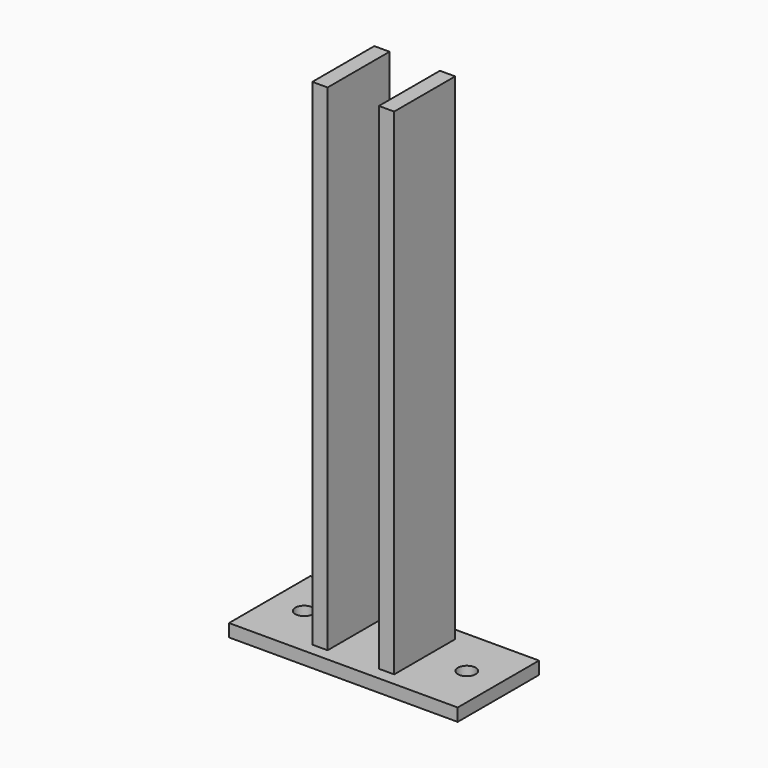
from build123d import *

# Parameters (mm, degrees)
F0_W     = 40
F0_H     = 5
F1_DEPTH = 90
F2_W     = 6
F2_H     = 30.4702166427
F2_H_2   = 30
F3_DEPTH = 200
F5_D     = 7


# Not quite as in the source:
# - a feature names something its author has since deleted; it is built from what else it names


with BuildPart() as f1:
    # F0 (on Right) → F1 (new body)
    with BuildSketch(Plane.YZ):
        with Locations((-0.72813743, 2.5)):
            Rectangle(F0_W, F0_H)
    extrude(amount=F1_DEPTH)

    # F2 (on Top) → F3 (join)
    with BuildSketch(Plane.XY):
        with Locations((32, -0.7447636027)):
            Rectangle(F2_W, F2_H)
        with Locations((58, -0.72813743)):
            Rectangle(F2_W, F2_H_2)
    extrude(amount=F3_DEPTH)

    # F5 (through all)
    with Locations(Plane(origin=(0, 0, 0), x_dir=(1, 0, 0), z_dir=(0, 0, -1))):
        with Locations((13, 0), (77, 0)):
            Hole(F5_D / 2)


solid = f1.part
